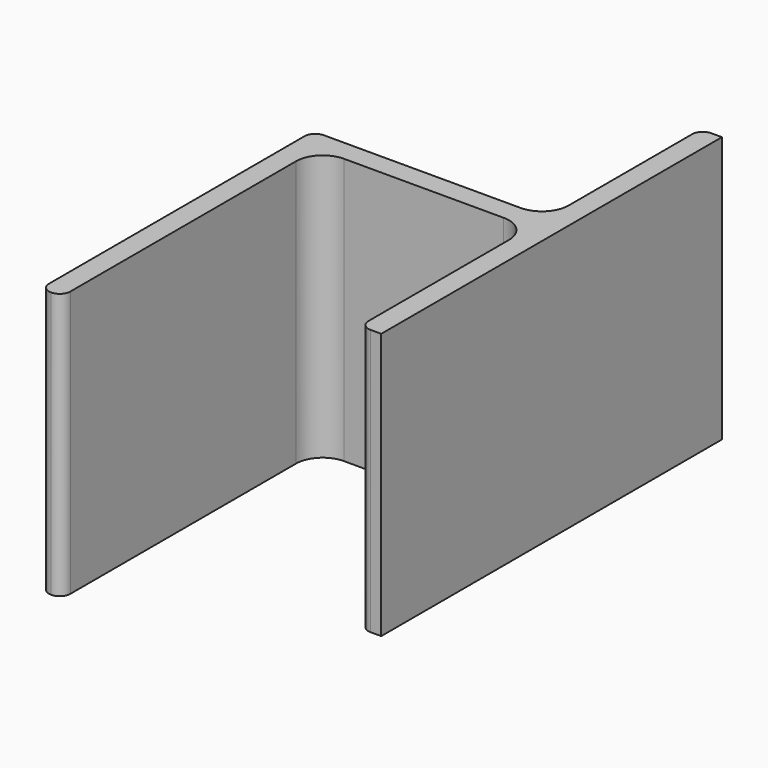
from build123d import *

# Parameters (mm, degrees)
F1_DEPTH      = 25
F2_DEPTH      = 25
F3_DEPTH      = 2
F3_DEPTH_BACK = 2
F4_R          = 5
F5_R          = 1.99999


# Not quite as in the source:
# - a fillet or chamfer is up to 0.001 mm smaller than in the source, because OpenCascade refuses the exact size


with BuildPart() as f1:
    # F0 (on Top) → F1 (new body)
    with BuildSketch(Plane.XY):
        Polygon((-40, 0), (-40, 4), (-44, 4), (-44, -60), (-40, -60), align=None)
        Polygon((0, 0), (0, 4), (-16, 4), (-40, 4), (-40, 0), align=None)
        Polygon((4, 40), (0, 40), (0, 29), (0, 4), (0, 0), (0, -40), (4, -40), align=None)
    extrude(amount=F1_DEPTH)

    # F0 (on Top) → F2 (join)
    with BuildSketch(Plane.XY):
        Polygon((4, 40), (0, 40), (0, 29), (0, 4), (0, 0), (0, -40), (4, -40), align=None)
        Polygon((0, 0), (0, 4), (-16, 4), (-40, 4), (-40, 0), align=None)
        Polygon((-40, 0), (-40, 4), (-44, 4), (-44, -60), (-40, -60), align=None)
    extrude(amount=-F2_DEPTH)

    # F0 (on Top) → F3 (join, two sides)
    with BuildSketch(Plane.XY) as f3_sk:
        Polygon((0, 4), (0, 29), (-16, 4), align=None)
    extrude(amount=F3_DEPTH)
    extrude(f3_sk.sketch, amount=-F3_DEPTH_BACK)

    # F4
    f4_edges = [f1.edges().sort_by_distance(p)[0] for p in [
        (-40, 0, 0),
        (0, 0, 0),
        (0, 4, 13.5),
        (0, 4, -13.5),
    ]]
    fillet(f4_edges, radius=F4_R)

    # F5 (radius 2 in the source; OpenCascade refuses exactly that, so slightly less here)
    f5_edges = [f1.edges().sort_by_distance(p)[0] for p in [
        (-44, 4, 0),
        (0, 40, 0),
        (-44, -60, 0),
        (-40, -60, 0),
        (0, -40, 0),
        (-16, 4, 0),
        (0, 29, 0),
    ]]
    fillet(f5_edges, radius=F5_R)


solid = f1.part
